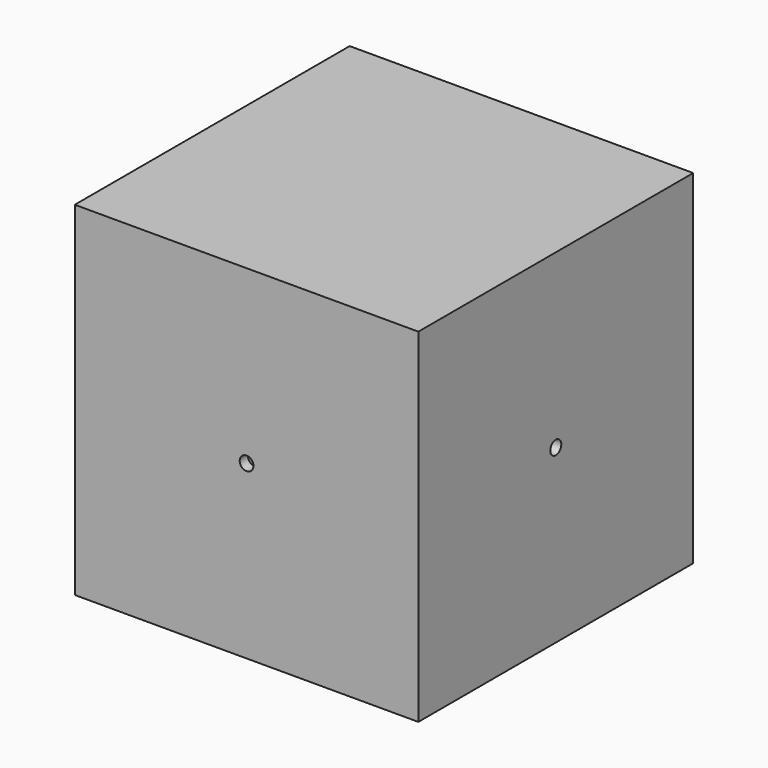
from build123d import *

# Parameters (mm, degrees)
F0_W     = 100
F0_H     = 100
F1_DEPTH = 100
F2_T     = -3
F3_R     = 2
F4_DEPTH = 100.001


# Not quite as in the source:
# - a pattern or mirror of a feature is missing from the dataset's text; its kind, count and spacing are read off the source's solid


with BuildPart() as f1:
    # F0 (on Top) → F1 (new body)
    with BuildSketch(Plane.XY):
        Rectangle(F0_W, F0_H)
    extrude(amount=F1_DEPTH)

    # F2 (hollow: no face is removed)
    offset(amount=F2_T, mode=Mode.SUBTRACT)

    # F3 (on face) → F4 (cut, through all)
    with BuildSketch(Plane(origin=(-50, 0, 0), x_dir=(0, -1, 0), z_dir=(-1, 0, 0))):
        with Locations((0, 50)):
            Circle(F3_R)
    f4 = extrude(amount=-F4_DEPTH, mode=Mode.SUBTRACT)

    # F4_copies: F4 across plane
    add(f4.mirror(Plane(origin=(0, 0, 0), x_dir=(0.7071067812, 0.7071067812, 0), z_dir=(-0.7071067812, 0.7071067812, 0))), mode=Mode.SUBTRACT)


solid = f1.part
